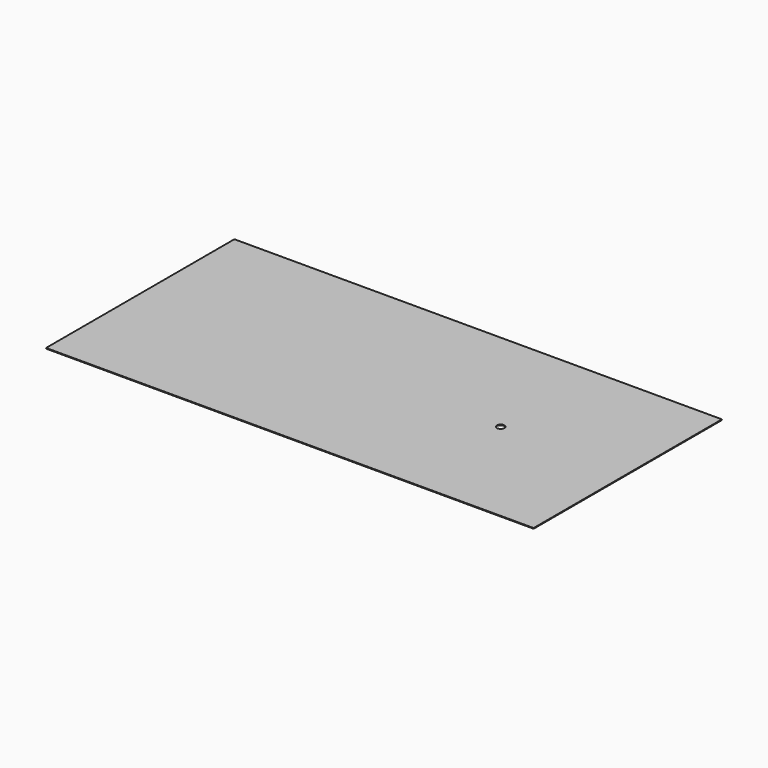
from build123d import *

# Parameters (mm, degrees)
F0_W           = 1450
F0_H           = 700
F1_DEPTH       = 2
F3_D           = 15.5
F3_DEPTH       = 14
F3_CBORE_D     = 22.25
F3_CBORE_DEPTH = 14
F3_TIP         = 4.6566697975


with BuildPart() as f1:
    # F0 (on Top) → F1 (new body)
    with BuildSketch(Plane.XY):
        with Locations((725, 350)):
            Rectangle(F0_W, F0_H)
    extrude(amount=F1_DEPTH)

    # F3
    with Locations(Plane.XY.offset(2)):
        with Locations((1072, 350)):
            CounterBoreHole(F3_D / 2, F3_CBORE_D / 2, F3_CBORE_DEPTH, depth=F3_DEPTH)
            with Locations((0, 0, -(F3_DEPTH + F3_TIP / 2))):  # 118° drill point
                Cone(0, F3_D / 2, F3_TIP, mode=Mode.SUBTRACT)


solid = f1.part
